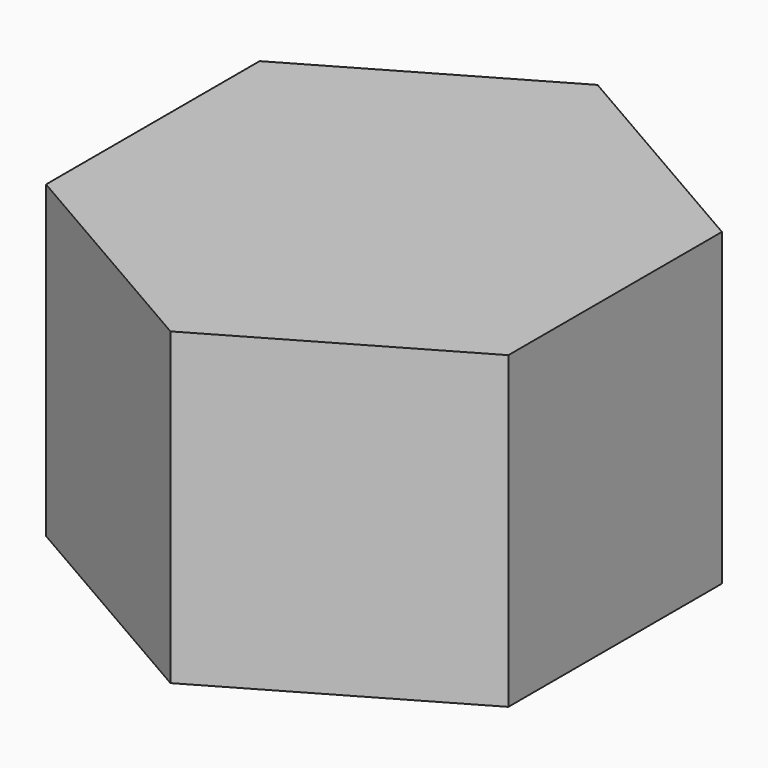
from build123d import *

# Parameters (mm, degrees)
F1_DEPTH = 6.35


# Not quite as in the source:
# - a feature names something its author has since deleted; it is built from what else it names


with BuildPart() as f1:
    # F0 (on Top) → F1 (new body)
    with BuildSketch(Plane.XY):
        Polygon((0, -5.4737), (4.7403632527, -2.73685), (4.7403632527, 2.73685), (0, 5.4737), (-4.7403632527, 2.73685), (-4.7403632527, -2.73685), align=None)
    extrude(amount=F1_DEPTH)


solid = f1.part
